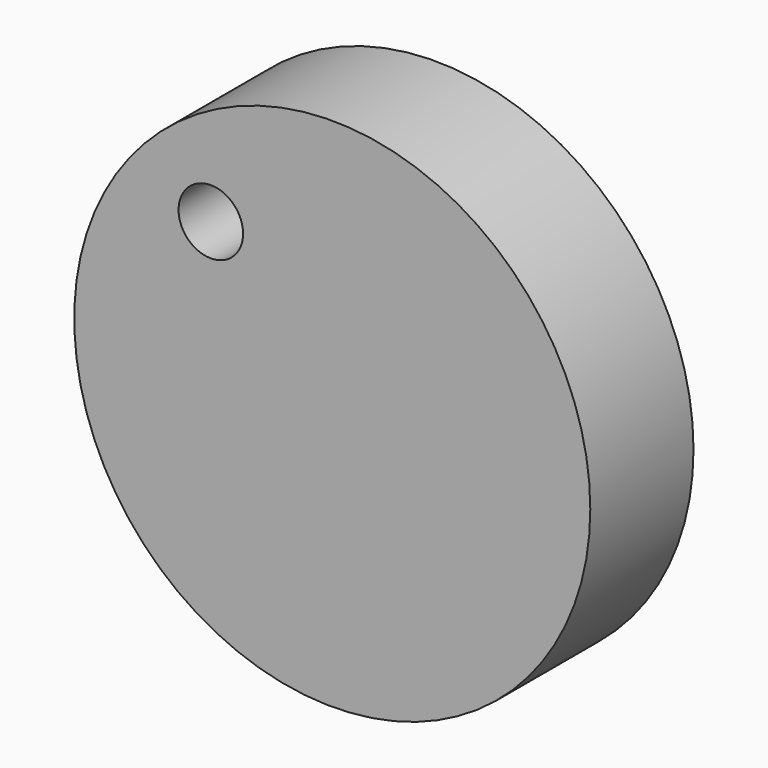
from build123d import *

# Parameters (mm, degrees)
F0_R     = 50.8
F0_R_2   = 6.35
F1_DEPTH = 25.4


# Not quite as in the source:
# - a feature of the source that left no trace in its solid (it failed there, or was rolled back) is left out


with BuildPart() as f1:
    # F0 (on Front) → F1 (new body)
    with BuildSketch(Plane.XZ):
        Circle(F0_R)
        with Locations((-23.9109713584, 25.5050305277)):
            Circle(F0_R_2, mode=Mode.SUBTRACT)
    extrude(amount=F1_DEPTH)


solid = f1.part
